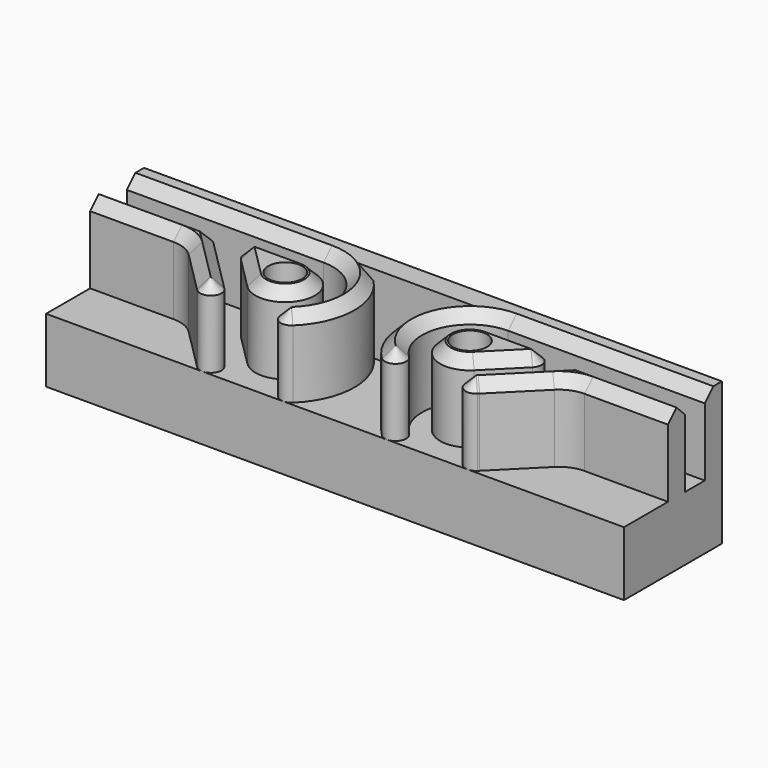
from build123d import *

# Parameters (mm, degrees)
F2_DEPTH     = 7.35
F1_R         = 1.6
F3_W         = 54
F3_H         = 11.4404760118
F3_R         = 1.6
F4_DEPTH     = 6
F5_T1_DEPTH  = 12.023863734
F5_T3_DEPTH  = 20.941682988
F5_T5_DEPTH  = 20.941682988
F5_T7_DEPTH  = 12.023863734
F5_T9_DEPTH  = 4.2852290732
F5_T11_DEPTH = 4.2852290732
F5_T13_DEPTH = 4.2852290732
F5_T15_DEPTH = 4.2852290732
F5_T17_DEPTH = 7.1367009358
F5_T19_DEPTH = 5.4798466863
F5_T21_DEPTH = 10.3670094845
F5_T23_DEPTH = 7.1367009358
F5_T25_DEPTH = 5.4798466863
F5_T27_DEPTH = 10.3670094845
F5_T30_ANGLE = 135
F5_T32_ANGLE = 225
F5_T34_ANGLE = 225
F5_T36_ANGLE = 135
F5_T38_ANGLE = 45
F5_T40_ANGLE = 1.4096380503
F5_T42_ANGLE = 180
F5_T44_ANGLE = 1.4096380503
F5_T46_ANGLE = 45
F5_T48_ANGLE = 136.4096380503
F5_T50_ANGLE = 180
F5_T54_ANGLE = 112.8938419293
F5_T57_ANGLE = 136.4096380503
F5_T59_ANGLE = 180
F5_T63_ANGLE = 112.8938419293
F5_T66_ANGLE = 45
F5_T68_ANGLE = 1.4096380503
F5_T70_ANGLE = 180
F5_T72_ANGLE = 1.4096380503
F5_T74_ANGLE = 45


# Not quite as in the source:
# - a fillet or chamfer that OpenCascade refuses, or shapes differently, is made with other operations: its cross-section is extruded or revolved along the edge and cut away or added


with BuildPart() as f2:
    # F1 (on offset) → F2 (new body)
    with BuildSketch(Plane.XY.offset(6)):
        with BuildLine():
            Line((27, 6.475), (-27, 6.475))
            Line((-27, 6.475), (-27, 4.475))
            Line((-27, 4.475), (-8.63, 4.475))
            ThreePointArc((-8.63, 4.475), (-4.474886163, 1.6615215923), (-5.5444977169, -3.2411881557))
            ThreePointArc((-5.5444977169, -3.2411881557), (-5.579287856, -4.6549737287), (-4.1655022831, -4.6897638678))
            ThreePointArc((-4.1655022831, -4.6897638678), (-2.1567850781, -0.1520314948), (-3.9502564173, 4.475))
            Line((-3.9502564173, 4.475), (3.9502564173, 4.475))
            ThreePointArc((3.9502564173, 4.475), (2.1567850781, -0.1520314948), (4.1655022831, -4.6897638678))
            ThreePointArc((4.1655022831, -4.6897638678), (5.579287856, -4.6549737287), (5.5444977169, -3.2411881557))
            ThreePointArc((5.5444977169, -3.2411881557), (4.474886163, 1.6615215923), (8.63, 4.475))
            Line((8.63, 4.475), (27, 4.475))
            Line((27, 4.475), (27, 6.475))
        make_face()
    extrude(amount=F2_DEPTH)



with BuildPart() as f2b:
    # F1 (on offset) → F2, piece 2 (new body)
    with BuildSketch(Plane.XY.offset(6)):
        with BuildLine():
            Line((-13.6223358544, 1.0678932188), (-10.5922213178, -1.9622213178))
            ThreePointArc((-10.5922213178, -1.9622213178), (-6.0662342973, -1.0619465248), (-8.63, 2.775))
            Line((-8.63, 2.775), (-12.9152290732, 2.775))
            ThreePointArc((-12.9152290732, 2.775), (-13.8391086057, 2.1576834324), (-13.6223358544, 1.0678932188))
        make_face()
        with Locations((-8.63, 0)):
            Circle(F1_R, mode=Mode.SUBTRACT)
    extrude(amount=F2_DEPTH)


with BuildPart() as f2c:
    # F1 (on offset) → F2, piece 3 (new body)
    with BuildSketch(Plane.XY.offset(6)):
        with BuildLine():
            ThreePointArc((8.63, 2.775), (6.0662342973, -1.0619465248), (10.5922213178, -1.9622213178))
            Line((10.5922213178, -1.9622213178), (13.6223358544, 1.0678932188))
            ThreePointArc((13.6223358544, 1.0678932188), (13.8391086057, 2.1576834324), (12.9152290732, 2.775))
            Line((12.9152290732, 2.775), (8.63, 2.775))
        make_face()
        with Locations((8.63, 0)):
            Circle(F1_R, mode=Mode.SUBTRACT)
    extrude(amount=F2_DEPTH)


with BuildPart() as f2d:
    # F1 (on offset) → F2, piece 4 (new body)
    with BuildSketch(Plane.XY.offset(6)):
        with BuildLine():
            Line((-17.547819254, 2.175), (-27, 2.175))
            Line((-27, 2.175), (-27, 0.175))
            Line((-27, 0.175), (-19.2046735035, 0.175))
            ThreePointArc((-19.2046735035, 0.175), (-18.0566232064, -0.0533614025), (-17.0833531599, -0.7036796564))
            Line((-17.0833531599, -0.7036796564), (-13.2085164082, -4.5785164082))
            ThreePointArc((-13.2085164082, -4.5785164082), (-13.1518491921, -4.6344907902), (-13.0944977169, -4.6897638678))
            ThreePointArc((-13.0944977169, -4.6897638678), (-11.680712144, -4.6549737287), (-11.7155022831, -3.2411881557))
            ThreePointArc((-11.7155022831, -3.2411881557), (-11.7551390169, -3.2029878434), (-11.7943028458, -3.1643028458))
            Line((-11.7943028458, -3.1643028458), (-16.8407124728, 1.8821067812))
            ThreePointArc((-16.8407124728, 1.8821067812), (-17.1651358216, 2.0988795325), (-17.547819254, 2.175))
        make_face()
    extrude(amount=F2_DEPTH)


with BuildPart() as f2e:
    # F1 (on offset) → F2, piece 5 (new body)
    with BuildSketch(Plane.XY.offset(6)):
        with BuildLine():
            ThreePointArc((13.0944977169, -4.6897638678), (13.1518491921, -4.6344907902), (13.2085164082, -4.5785164082))
            Line((13.2085164082, -4.5785164082), (17.0833531599, -0.7036796564))
            ThreePointArc((17.0833531599, -0.7036796564), (18.0566232064, -0.0533614025), (19.2046735035, 0.175))
            Line((19.2046735035, 0.175), (27, 0.175))
            Line((27, 0.175), (27, 2.175))
            Line((27, 2.175), (17.547819254, 2.175))
            ThreePointArc((17.547819254, 2.175), (17.1651358216, 2.0988795325), (16.8407124728, 1.8821067812))
            Line((16.8407124728, 1.8821067812), (11.7943028458, -3.1643028458))
            ThreePointArc((11.7943028458, -3.1643028458), (11.7551390169, -3.2029878434), (11.7155022831, -3.2411881557))
            ThreePointArc((11.7155022831, -3.2411881557), (11.680712144, -4.6549737287), (13.0944977169, -4.6897638678))
        make_face()
    extrude(amount=F2_DEPTH)


with BuildPart() as f2_1:
    add(f2.part)

    add(f2b.part)  # F4 merges F2b

    add(f2c.part)  # F4 merges F2c

    add(f2d.part)  # F4 merges F2d

    add(f2e.part)  # F4 merges F2e
    # F3 (on face) → F4 (join, through all)
    with BuildSketch(Plane(origin=(0, 0, 6), x_dir=(1, 0, 0), z_dir=(0, 0, -1))):
        with Locations((0, -0.7547619941)):
            Rectangle(F3_W, F3_H)
        with Locations((-8.63, 0)):
            Circle(F3_R, mode=Mode.SUBTRACT)
        with Locations((8.63, 0)):
            Circle(F3_R, mode=Mode.SUBTRACT)
    extrude(amount=F4_DEPTH)

    # F5: chamfer of 1 on 6 edges, made by hand

    # F5_s2 → F5_t1 (cut)
    with BuildSketch(Plane.YZ.offset(-29.571682988)):
        Polygon((2.175, 12.35), (1.175, 13.35), (2.175, 13.35), align=None)
    extrude(amount=F5_T1_DEPTH, mode=Mode.SUBTRACT)

    # F5_s4 → F5_t3 (cut)
    with BuildSketch(Plane.YZ.offset(-29.571682988)):
        Polygon((5.475, 13.35), (4.475, 12.35), (4.475, 13.35), align=None)
    extrude(amount=F5_T3_DEPTH, mode=Mode.SUBTRACT)

    # F5_s6 → F5_t5 (cut)
    with BuildSketch(Plane.YZ.offset(8.63)):
        Polygon((4.475, 12.35), (5.475, 13.35), (4.475, 13.35), align=None)
    extrude(amount=F5_T5_DEPTH, mode=Mode.SUBTRACT)

    # F5_s8 → F5_t7 (cut)
    with BuildSketch(Plane.YZ.offset(17.547819254)):
        Polygon((1.175, 13.35), (2.175, 12.35), (2.175, 13.35), align=None)
    extrude(amount=F5_T7_DEPTH, mode=Mode.SUBTRACT)

    # F5_s10 → F5_t9 (cut)
    with BuildSketch(Plane.YZ.offset(-12.9152290732)):
        Polygon((2.775, 12.35), (1.775, 13.35), (2.775, 13.35), align=None)
    extrude(amount=F5_T9_DEPTH, mode=Mode.SUBTRACT)

    # F5_s12 → F5_t11 (cut)
    with BuildSketch(Plane.YZ.offset(8.63)):
        Polygon((2.775, 12.35), (1.775, 13.35), (2.775, 13.35), align=None)
    extrude(amount=F5_T11_DEPTH, mode=Mode.SUBTRACT)

    # F5_s14 → F5_t13 (cut)
    with BuildSketch(Plane(origin=(4.315, 4.315, 0), x_dir=(0, 0, 1), z_dir=(0.7071067812, 0.7071067812, 0))):
        Polygon((12.35, 8.8773315216), (13.35, 7.8773315216), (13.35, 8.8773315216), align=None)
    extrude(amount=F5_T13_DEPTH, mode=Mode.SUBTRACT)

    # F5_s16 → F5_t15 (cut)
    with BuildSketch(Plane(origin=(-7.3451145366, 7.3451145366, 0), x_dir=(0, 0, 1), z_dir=(0.7071067812, -0.7071067812, 0))):
        Polygon((12.35, 8.8773315216), (13.35, 7.8773315216), (13.35, 8.8773315216), align=None)
    extrude(amount=F5_T15_DEPTH, mode=Mode.SUBTRACT)

    # F5_s18 → F5_t17 (cut)
    with BuildSketch(Plane(origin=(9.361409627, 9.361409627, 0), x_dir=(0, 0, 1), z_dir=(-0.7071067812, -0.7071067812, 0))):
        Polygon((13.35, -11.5773315216), (12.35, -10.5773315216), (13.35, -10.5773315216), align=None)
    extrude(amount=F5_T17_DEPTH, mode=Mode.SUBTRACT)

    # F5_s20 → F5_t19 (cut)
    with BuildSketch(Plane(origin=(4.315, 4.315, 0), x_dir=(0, 0, 1), z_dir=(0.7071067812, 0.7071067812, 0))):
        Polygon((13.35, 11.5773315216), (12.35, 12.5773315216), (13.35, 12.5773315216), align=None)
    extrude(amount=F5_T19_DEPTH, mode=Mode.SUBTRACT)

    # F5_s22 → F5_t21 (cut)
    with BuildSketch(Plane.YZ.offset(19.2046735035)):
        Polygon((1.175, 13.35), (0.175, 12.35), (0.175, 13.35), align=None)
    extrude(amount=F5_T21_DEPTH, mode=Mode.SUBTRACT)

    # F5_s24 → F5_t23 (cut)
    with BuildSketch(Plane(origin=(-4.315, 4.315, 0), x_dir=(0, 0, 1), z_dir=(-0.7071067812, 0.7071067812, 0))):
        Polygon((13.35, -11.5773315216), (12.35, -10.5773315216), (13.35, -10.5773315216), align=None)
    extrude(amount=F5_T23_DEPTH, mode=Mode.SUBTRACT)

    # F5_s26 → F5_t25 (cut)
    with BuildSketch(Plane(origin=(-8.1898367517, 8.1898367517, 0), x_dir=(0, 0, 1), z_dir=(0.7071067812, -0.7071067812, 0))):
        Polygon((13.35, 11.5773315216), (12.35, 12.5773315216), (13.35, 12.5773315216), align=None)
    extrude(amount=F5_T25_DEPTH, mode=Mode.SUBTRACT)

    # F5_s28 → F5_t27 (cut)
    with BuildSketch(Plane.YZ.offset(-29.571682988)):
        Polygon((1.175, 13.35), (0.175, 12.35), (0.175, 13.35), align=None)
    extrude(amount=F5_T27_DEPTH, mode=Mode.SUBTRACT)

    # F5_s29 → F5_t30 (revolve, cut)
    with BuildSketch(Plane(origin=(7.3451145366, 7.3451145366, 0), x_dir=(0, 0, 1), z_dir=(-0.7071067812, -0.7071067812, 0))):
        Polygon((12.35, -8.8773315216), (13.35, -7.8773315216), (13.35, -8.8773315216), align=None)
    revolve(axis=Axis((12.9152290732, 1.775, 13.35), (0, 0, 1)), revolution_arc=F5_T30_ANGLE, mode=Mode.SUBTRACT)

    # F5_s31 → F5_t32 (revolve, cut)
    with BuildSketch(Plane.YZ.offset(8.63)):
        Polygon((2.775, 12.35), (1.775, 13.35), (2.775, 13.35), align=None)
    revolve(axis=Axis((8.63, 0, 13.35), (0, 0, 1)), revolution_arc=F5_T32_ANGLE, mode=Mode.SUBTRACT)

    # F5_s33 → F5_t34 (revolve, cut)
    with BuildSketch(Plane(origin=(-4.315, 4.315, 0), x_dir=(0, 0, 1), z_dir=(-0.7071067812, 0.7071067812, 0))):
        Polygon((12.35, -8.8773315216), (13.35, -7.8773315216), (13.35, -8.8773315216), align=None)
    revolve(axis=Axis((-8.63, 0, 13.35), (0, 0, 1)), revolution_arc=F5_T34_ANGLE, mode=Mode.SUBTRACT)

    # F5_s35 → F5_t36 (revolve, cut)
    with BuildSketch(Plane.YZ.offset(-12.9152290732)):
        Polygon((2.775, 12.35), (1.775, 13.35), (2.775, 13.35), align=None)
    revolve(axis=Axis((-12.9152290732, 1.775, 13.35), (0, 0, 1)), revolution_arc=F5_T36_ANGLE, mode=Mode.SUBTRACT)

    # F5_s37 → F5_t38 (revolve, cut)
    with BuildSketch(Plane.YZ.offset(17.547819254)):
        Polygon((1.175, 13.35), (2.175, 12.35), (2.175, 13.35), align=None)
    revolve(axis=Axis((17.547819254, 1.175, 13.35), (0, 0, 1)), revolution_arc=F5_T38_ANGLE, mode=Mode.SUBTRACT)

    # F5_s39 → F5_t40 (revolve, cut)
    with BuildSketch(Plane(origin=(4.315, 4.315, 0), x_dir=(0, 0, 1), z_dir=(0.7071067812, 0.7071067812, 0))):
        Polygon((12.35, 10.5773315216), (13.35, 11.5773315216), (13.35, 10.5773315216), align=None)
    revolve(axis=Axis((8.63, 0, 13.35), (0, 0, -1)), revolution_arc=F5_T40_ANGLE, mode=Mode.SUBTRACT)

    # F5_s41 → F5_t42 (revolve, cut)
    with BuildSketch(Plane(origin=(4.5272367132, 4.3097773234, 0), x_dir=(0, 0, 1), z_dir=(0.724287856, 0.6894977169, 0))):
        Polygon((12.35, 10.4253652968), (13.35, 11.4253652968), (13.35, 10.4253652968), align=None)
    revolve(axis=Axis((12.405, -3.9654760118, 13.35), (0, 0, 1)), revolution_arc=F5_T42_ANGLE, mode=Mode.SUBTRACT)

    # F5_s43 → F5_t44 (revolve, cut)
    with BuildSketch(Plane(origin=(4.5272367132, 4.3097773234, 0), x_dir=(0, 0, 1), z_dir=(-0.724287856, -0.6894977169, 0))):
        Polygon((12.35, -12.4253652968), (13.35, -11.4253652968), (13.35, -12.4253652968), align=None)
    revolve(axis=Axis((8.63, 0, 13.35), (0, 0, 1)), revolution_arc=F5_T44_ANGLE, mode=Mode.SUBTRACT)

    # F5_s45 → F5_t46 (revolve, cut)
    with BuildSketch(Plane(origin=(8.1898367517, 8.1898367517, 0), x_dir=(0, 0, 1), z_dir=(-0.7071067812, -0.7071067812, 0))):
        Polygon((13.35, -11.5773315216), (12.35, -12.5773315216), (13.35, -12.5773315216), align=None)
    revolve(axis=Axis((19.2046735035, -2.825, 13.35), (0, 0, -1)), revolution_arc=F5_T46_ANGLE, mode=Mode.SUBTRACT)

    # F5_s47 → F5_t48 (revolve, cut)
    with BuildSketch(Plane(origin=(4.5272367132, -4.3097773234, 0), x_dir=(0, 0, 1), z_dir=(0.724287856, -0.6894977169, 0))):
        Polygon((12.35, -1.4753652968), (13.35, -0.4753652968), (13.35, -1.4753652968), align=None)
    revolve(axis=Axis((8.63, 0, 13.35), (0, 0, -1)), revolution_arc=F5_T48_ANGLE, mode=Mode.SUBTRACT)

    # F5_s49 → F5_t50 (revolve, cut)
    with BuildSketch(Plane(origin=(4.5272367132, -4.3097773234, 0), x_dir=(0, 0, 1), z_dir=(-0.724287856, 0.6894977169, 0))):
        Polygon((12.35, -0.5246347032), (13.35, 0.4753652968), (13.35, -0.5246347032), align=None)
    revolve(axis=Axis((4.855, -3.9654760118, 13.35), (0, 0, 1)), revolution_arc=F5_T50_ANGLE, mode=Mode.SUBTRACT)


with BuildPart() as f5_tool52:
    # F5_s53 → F5_t54 (revolve)
    with BuildSketch(Plane(origin=(7.256082409, 3.1574133818, 0), x_dir=(0, 0, 1), z_dir=(0.9169501067, 0.399001882, 0))):
        Polygon((13.35, -2.0316137581), (12.35, -3.0316137581), (13.35, -3.0316137581), align=None)
    revolve(axis=Axis((8.63, 0, 13.35), (0, 0, 1)), revolution_arc=F5_T54_ANGLE)

    split(bisect_by=Plane.XZ.offset(-4.475), keep=Keep.TOP)


with BuildPart() as f2_2:
    add(f2_1.part)

    # F5_t51: cut F5_tool52
    add(f5_tool52.part, mode=Mode.SUBTRACT)

    # F5_s56 → F5_t57 (revolve, cut)
    with BuildSketch(Plane.YZ.offset(-8.63)):
        Polygon((5.475, 13.35), (4.475, 12.35), (4.475, 13.35), align=None)
    revolve(axis=Axis((-8.63, 0, 13.35), (0, 0, -1)), revolution_arc=F5_T57_ANGLE, mode=Mode.SUBTRACT)

    # F5_s58 → F5_t59 (revolve, cut)
    with BuildSketch(Plane(origin=(-4.5272367132, -4.3097773234, 0), x_dir=(0, 0, 1), z_dir=(0.724287856, 0.6894977169, 0))):
        Polygon((13.35, -0.4753652968), (12.35, -1.4753652968), (13.35, -1.4753652968), align=None)
    revolve(axis=Axis((-4.855, -3.9654760118, 13.35), (0, 0, 1)), revolution_arc=F5_T59_ANGLE, mode=Mode.SUBTRACT)


with BuildPart() as f5_tool61:
    # F5_s62 → F5_t63 (revolve)
    with BuildSketch(Plane(origin=(-4.5272367132, -4.3097773234, 0), x_dir=(0, 0, 1), z_dir=(-0.724287856, -0.6894977169, 0))):
        Polygon((13.35, 0.4753652968), (12.35, -0.5246347032), (13.35, -0.5246347032), align=None)
    revolve(axis=Axis((-8.63, 0, 13.35), (0, 0, 1)), revolution_arc=F5_T63_ANGLE)

    split(bisect_by=Plane.XZ.offset(-4.475), keep=Keep.TOP)


with BuildPart() as f2_3:
    add(f2_2.part)

    # F5_t60: cut F5_tool61
    add(f5_tool61.part, mode=Mode.SUBTRACT)

    # F5_s65 → F5_t66 (revolve, cut)
    with BuildSketch(Plane(origin=(-9.361409627, 9.361409627, 0), x_dir=(0, 0, 1), z_dir=(0.7071067812, -0.7071067812, 0))):
        Polygon((13.35, 11.5773315216), (12.35, 10.5773315216), (13.35, 10.5773315216), align=None)
    revolve(axis=Axis((-17.547819254, 1.175, 13.35), (0, 0, 1)), revolution_arc=F5_T66_ANGLE, mode=Mode.SUBTRACT)

    # F5_s67 → F5_t68 (revolve, cut)
    with BuildSketch(Plane(origin=(-4.5272367132, 4.3097773234, 0), x_dir=(0, 0, 1), z_dir=(0.724287856, -0.6894977169, 0))):
        Polygon((13.35, 11.4253652968), (12.35, 10.4253652968), (13.35, 10.4253652968), align=None)
    revolve(axis=Axis((-8.63, 0, 13.35), (0, 0, -1)), revolution_arc=F5_T68_ANGLE, mode=Mode.SUBTRACT)

    # F5_s69 → F5_t70 (revolve, cut)
    with BuildSketch(Plane(origin=(-4.5272367132, 4.3097773234, 0), x_dir=(0, 0, 1), z_dir=(-0.724287856, 0.6894977169, 0))):
        Polygon((13.35, -11.4253652968), (12.35, -12.4253652968), (13.35, -12.4253652968), align=None)
    revolve(axis=Axis((-12.405, -3.9654760118, 13.35), (0, 0, 1)), revolution_arc=F5_T70_ANGLE, mode=Mode.SUBTRACT)

    # F5_s71 → F5_t72 (revolve, cut)
    with BuildSketch(Plane(origin=(-4.315, 4.315, 0), x_dir=(0, 0, 1), z_dir=(-0.7071067812, 0.7071067812, 0))):
        Polygon((13.35, -11.5773315216), (12.35, -12.5773315216), (13.35, -12.5773315216), align=None)
    revolve(axis=Axis((-8.63, 0, 13.35), (0, 0, 1)), revolution_arc=F5_T72_ANGLE, mode=Mode.SUBTRACT)

    # F5_s73 → F5_t74 (revolve, cut)
    with BuildSketch(Plane.YZ.offset(-19.2046735035)):
        Polygon((1.175, 13.35), (0.175, 12.35), (0.175, 13.35), align=None)
    revolve(axis=Axis((-19.2046735035, -2.825, 13.35), (0, 0, -1)), revolution_arc=F5_T74_ANGLE, mode=Mode.SUBTRACT)


solid = f2_3.part
